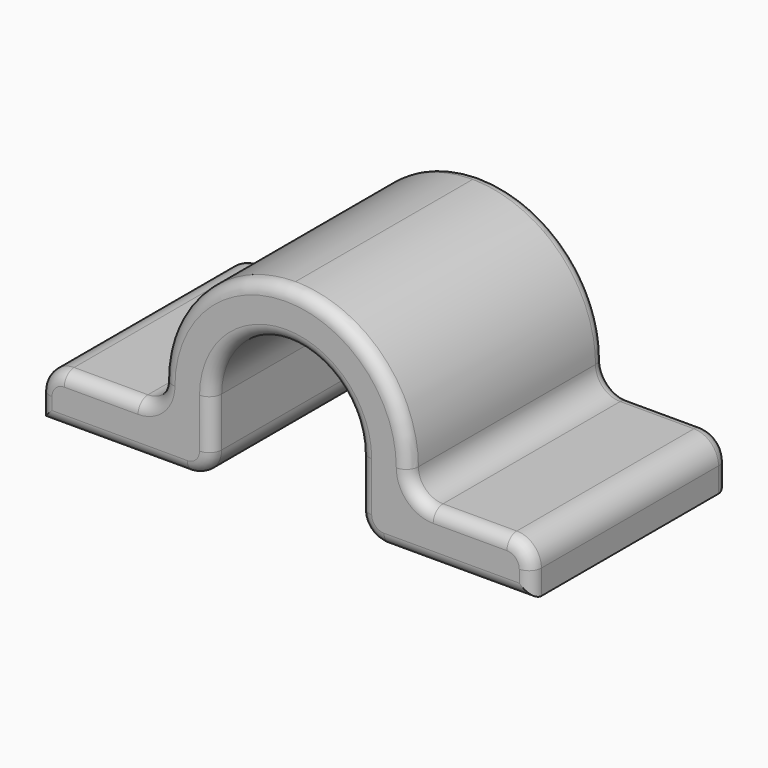
from build123d import *

# Parameters (mm, degrees)
F1_DEPTH     = 10
F2_R         = 0.99999
F3_T1_DEPTH  = 1e-05
F3_T3_DEPTH  = 2.00001
F3_T5_DEPTH  = 7.25001
F3_T7_DEPTH  = 3.00002
F3_T9_DEPTH  = 2.25001
F3_T12_ANGLE = 113.8828315396
F3_T14_ANGLE = 104.3296989237
F3_T16_ANGLE = 90
F3_T18_ANGLE = 113.8828315396
F3_T20_ANGLE = 90
F3_T22_ANGLE = 104.3296989237
F3_T24_ANGLE = 90
F3_T26_ANGLE = 90
F3_T28_ANGLE = 90
F3_T30_ANGLE = 90


# Not quite as in the source:
# - a fillet or chamfer that OpenCascade refuses, or shapes differently, is made with other operations: its cross-section is extruded or revolved along the edge and cut away or added
# - a fillet or chamfer is up to 0.001 mm smaller than in the source, because OpenCascade refuses the exact size


with BuildPart() as f1:
    # F0 (on Front) → F1 (new body)
    with BuildSketch(Plane.XZ):
        with BuildLine():
            Line((5, 2), (5, 3))
            ThreePointArc((5, 3), (4.7434164903, 1.4188611699), (4, 0))
            Line((4, 0), (5, 0))
            Line((5, 0), (10, 0))
            Line((10, 0), (10, 2))
            Line((10, 2), (5, 2))
        make_face()
        with BuildLine():
            Line((5, 3), (3, 3))
            Line((3, 3), (3, 0))
            Line((3, 0), (4, 0))
            ThreePointArc((4, 0), (4.7434164903, 1.4188611699), (5, 3))
        make_face()
        with BuildLine():
            Line((0, 8), (0, 6))
            ThreePointArc((0, 6), (2.1213203436, 5.1213203436), (3, 3))
            Line((3, 3), (5, 3))
            ThreePointArc((5, 3), (3.5355339059, 6.5355339059), (0, 8))
        make_face()
    extrude(amount=F1_DEPTH)

    # F2 (radius 1 in the source; OpenCascade refuses exactly that, so slightly less here)
    f2_edges = [f1.edges().sort_by_distance(p)[0] for p in [
        (5, -5, 2),
        (3, -5, 0),
        (10, -5, 2),
    ]]
    fillet(f2_edges, radius=F2_R)

    # F3: fillet of radius 0.5 on 5 edges, made by hand

    # F3_s2 → F3_t1 (cut)
    with BuildSketch(Plane.XY.offset(2.99999)):
        with BuildLine():
            ThreePointArc((4.5, -10), (4.8535533906, -9.8535533906), (5, -9.5))
            Line((5, -9.5), (5, -10))
            Line((5, -10), (4.5, -10))
        make_face()
        with BuildLine():
            ThreePointArc((4.5, 0), (4.8535533906, -0.1464466094), (5, -0.5))
            Line((5, -0.5), (5, 0))
            Line((5, 0), (4.5, 0))
        make_face()
    extrude(amount=F3_T1_DEPTH, mode=Mode.SUBTRACT)

    # F3_s4 → F3_t3 (cut)
    with BuildSketch(Plane.XY.offset(0.99999)):
        with BuildLine():
            ThreePointArc((3.5, 0), (3.1464466094, -0.1464466094), (3, -0.5))
            Line((3, -0.5), (3, 0))
            Line((3, 0), (3.5, 0))
        make_face()
        with BuildLine():
            ThreePointArc((3.5, -10), (3.1464466094, -9.8535533906), (3, -9.5))
            Line((3, -9.5), (3, -10))
            Line((3, -10), (3.5, -10))
        make_face()
    extrude(amount=F3_T3_DEPTH, mode=Mode.SUBTRACT)

    # F3_s6 → F3_t5 (cut)
    with BuildSketch(Plane.YZ.offset(3.99999)):
        with BuildLine():
            ThreePointArc((0, 0.5), (-0.1464466094, 0.1464466094), (-0.5, 0))
            Line((-0.5, 0), (0, 0))
            Line((0, 0), (0, 0.5))
        make_face()
        with BuildLine():
            ThreePointArc((-9.5, 0), (-9.8535533906, 0.1464466094), (-10, 0.5))
            Line((-10, 0.5), (-10, 0))
            Line((-10, 0), (-9.5, 0))
        make_face()
    extrude(amount=F3_T5_DEPTH, mode=Mode.SUBTRACT)

    # F3_s8 → F3_t7 (cut)
    with BuildSketch(Plane.YZ.offset(5.99999)):
        with BuildLine():
            ThreePointArc((0, 1.5), (-0.1464466094, 1.8535533906), (-0.5, 2))
            Line((-0.5, 2), (0, 2))
            Line((0, 2), (0, 1.5))
        make_face()
        with BuildLine():
            ThreePointArc((-10, 1.5), (-9.8535533906, 1.8535533906), (-9.5, 2))
            Line((-9.5, 2), (-10, 2))
            Line((-10, 2), (-10, 1.5))
        make_face()
    extrude(amount=F3_T7_DEPTH, mode=Mode.SUBTRACT)

    # F3_s10 → F3_t9 (cut)
    with BuildSketch(Plane.XY.offset(-1.25)):
        with BuildLine():
            ThreePointArc((10, -0.5), (9.8535533906, -0.1464466094), (9.5, 0))
            Line((9.5, 0), (10, 0))
            Line((10, 0), (10, -0.5))
        make_face()
        with BuildLine():
            ThreePointArc((10, -9.5), (9.8535533906, -9.8535533906), (9.5, -10))
            Line((9.5, -10), (10, -10))
            Line((10, -10), (10, -9.5))
        make_face()
    extrude(amount=F3_T9_DEPTH, mode=Mode.SUBTRACT)

    # F3_s11 → F3_t12 (revolve, cut)
    with BuildSketch(Plane(origin=(1.1106028594, 0, 0.4917533592), x_dir=(0, 1, 0), z_dir=(-0.9143753133, 0, -0.4048676159))):
        with BuildLine():
            ThreePointArc((-10, -6.2431259399), (-9.8535533906, -5.8895725493), (-9.5, -5.7431259399))
            Line((-9.5, -5.7431259399), (-10, -5.7431259399))
            Line((-10, -5.7431259399), (-10, -6.2431259399))
        make_face()
    revolve(axis=Axis((0, -10, 3), (0, 1, 0)), revolution_arc=F3_T12_ANGLE, mode=Mode.SUBTRACT)

    # F3_s13 → F3_t14 (revolve, cut)
    with BuildSketch(Plane.XY.offset(3)):
        with BuildLine():
            ThreePointArc((4.5, -10), (4.8535533906, -9.8535533906), (5, -9.5))
            Line((5, -9.5), (5, -10))
            Line((5, -10), (4.5, -10))
        make_face()
    revolve(axis=Axis((0, -10, 3), (0, -1, 0)), revolution_arc=F3_T14_ANGLE, mode=Mode.SUBTRACT)

    # F3_s15 → F3_t16 (revolve, cut)
    with BuildSketch(Plane.YZ.offset(5.99999)):
        with BuildLine():
            ThreePointArc((0, 1.5), (-0.1464466094, 1.8535533906), (-0.5, 2))
            Line((-0.5, 2), (0, 2))
            Line((0, 2), (0, 1.5))
        make_face()
    revolve(axis=Axis((5.99999, 0, 2.99999), (0, 1, 0)), revolution_arc=F3_T16_ANGLE, mode=Mode.SUBTRACT)

    # F3_s17 → F3_t18 (revolve, cut)
    with BuildSketch(Plane(origin=(1.1106028594, 0, 0.4917533592), x_dir=(0, 1, 0), z_dir=(-0.9143753133, 0, -0.4048676159))):
        with BuildLine():
            ThreePointArc((0, -6.2431259399), (-0.1464466094, -5.8895725493), (-0.5, -5.7431259399))
            Line((-0.5, -5.7431259399), (0, -5.7431259399))
            Line((0, -5.7431259399), (0, -6.2431259399))
        make_face()
    revolve(axis=Axis((0, 0, 3), (0, 1, 0)), revolution_arc=F3_T18_ANGLE, mode=Mode.SUBTRACT)

    # F3_s19 → F3_t20 (revolve, cut)
    with BuildSketch(Plane.XY.offset(0.99999)):
        with BuildLine():
            ThreePointArc((3.5, 0), (3.1464466094, -0.1464466094), (3, -0.5))
            Line((3, -0.5), (3, 0))
            Line((3, 0), (3.5, 0))
        make_face()
    revolve(axis=Axis((3.99999, 0, 0.99999), (0, -1, 0)), revolution_arc=F3_T20_ANGLE, mode=Mode.SUBTRACT)

    # F3_s21 → F3_t22 (revolve, cut)
    with BuildSketch(Plane.XY.offset(3)):
        with BuildLine():
            ThreePointArc((4.5, 0), (4.8535533906, -0.1464466094), (5, -0.5))
            Line((5, -0.5), (5, 0))
            Line((5, 0), (4.5, 0))
        make_face()
    revolve(axis=Axis((0, 0, 3), (0, -1, 0)), revolution_arc=F3_T22_ANGLE, mode=Mode.SUBTRACT)

    # F3_s23 → F3_t24 (revolve, cut)
    with BuildSketch(Plane.XY.offset(1.00001)):
        with BuildLine():
            ThreePointArc((9.5, 0), (9.8535533906, -0.1464466094), (10, -0.5))
            Line((10, -0.5), (10, 0))
            Line((10, 0), (9.5, 0))
        make_face()
    revolve(axis=Axis((9.00001, 0, 1.00001), (0, -1, 0)), revolution_arc=F3_T24_ANGLE, mode=Mode.SUBTRACT)

    # F3_s25 → F3_t26 (revolve, cut)
    with BuildSketch(Plane.YZ.offset(5.99999)):
        with BuildLine():
            ThreePointArc((-10, 1.5), (-9.8535533906, 1.8535533906), (-9.5, 2))
            Line((-9.5, 2), (-10, 2))
            Line((-10, 2), (-10, 1.5))
        make_face()
    revolve(axis=Axis((5.99999, -10, 2.99999), (0, 1, 0)), revolution_arc=F3_T26_ANGLE, mode=Mode.SUBTRACT)

    # F3_s27 → F3_t28 (revolve, cut)
    with BuildSketch(Plane.XY.offset(1.00001)):
        with BuildLine():
            ThreePointArc((10, -9.5), (9.8535533906, -9.8535533906), (9.5, -10))
            Line((9.5, -10), (10, -10))
            Line((10, -10), (10, -9.5))
        make_face()
    revolve(axis=Axis((9.00001, -10, 1.00001), (0, -1, 0)), revolution_arc=F3_T28_ANGLE, mode=Mode.SUBTRACT)

    # F3_s29 → F3_t30 (revolve, cut)
    with BuildSketch(Plane.XY.offset(0.99999)):
        with BuildLine():
            ThreePointArc((3.5, -10), (3.1464466094, -9.8535533906), (3, -9.5))
            Line((3, -9.5), (3, -10))
            Line((3, -10), (3.5, -10))
        make_face()
    revolve(axis=Axis((3.99999, -10, 0.99999), (0, -1, 0)), revolution_arc=F3_T30_ANGLE, mode=Mode.SUBTRACT)

    # F4: F1 across face


with BuildPart() as f1_1:
    add(f1.part)
    add(f1.part.mirror(Plane(origin=(0, -5, 7), x_dir=(0, -1, 0), z_dir=(-1, 0, 0))))


solid = f1_1.part
